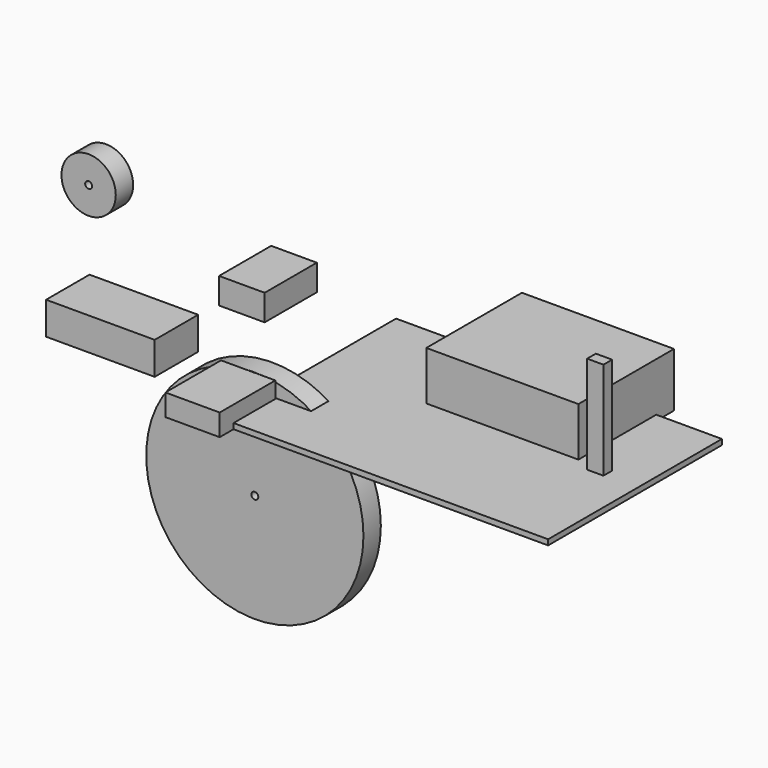
from build123d import *

# Parameters (mm, degrees)
F0_W      = 50
F0_H      = 25
F1_DEPTH  = 15
F2_W      = 70
F2_H      = 55
F3_DEPTH  = 25
F4_W      = 21
F4_H      = 12
F5_DEPTH  = 30
F6_W      = 25
F6_H      = 32
F7_DEPTH  = 10
F8_W      = 150
F8_H      = 100
F9_DEPTH  = 2.5
F10_R     = 50
F10_R_2   = 1.5875
F11_DEPTH = 10
F12_R     = 12.5
F12_R_2   = 1.5875
F13_DEPTH = 10
F14_W     = 7.5
F14_H     = 44.9961
F15_DEPTH = 5


# Not quite as in the source:
# - a feature names something its author has since deleted; it is built from what else it names


with BuildPart() as f1:
    # F0 (on Top) → F1 (new body)
    with BuildSketch(Plane.XY):
        with Locations((-111.7799058557, -7.9904274056)):
            Rectangle(F0_W, F0_H)
    extrude(amount=F1_DEPTH)


with BuildPart() as f3:
    # F2 (on Top) → F3 (new body)
    with BuildSketch(Plane.XY):
        with Locations((40.3834730387, 48.0927660437)):
            Rectangle(F2_W, F2_H)
    extrude(amount=F3_DEPTH)


with BuildPart() as f5:
    # F4 (on Front) → F5 (new body)
    with BuildSketch(Plane.XZ):
        with Locations((-39.0541495681, 50.8754973734)):
            Rectangle(F4_W, F4_H)
    extrude(amount=F5_DEPTH)


with BuildPart() as f7:
    # F6 (on Top) → F7 (new body)
    with BuildSketch(Plane.XY):
        with Locations((-51.6924057156, -26.56879695)):
            Rectangle(F6_W, F6_H)
    extrude(amount=F7_DEPTH)


with BuildPart() as f9:
    # F8 (on Top) → F9 (new body)
    with BuildSketch(Plane.XY):
        with Locations((30.6242685765, 15.3774665831)):
            Rectangle(F8_W, F8_H)
    extrude(amount=F9_DEPTH)


with BuildPart() as f11:
    # F10 (on Front) → F11 (new body)
    with BuildSketch(Plane.XZ):
        with Locations((-49.077399075, -40.1809364557)):
            Circle(F10_R)
        with Locations((-49.077399075, -40.1809364557)):
            Circle(F10_R_2, mode=Mode.SUBTRACT)
    extrude(amount=F11_DEPTH)


with BuildPart() as f13:
    # F12 (on Front) → F13 (new body)
    with BuildSketch(Plane.XZ):
        with Locations((-125.5905777216, 60.8639121056)):
            Circle(F12_R)
        with Locations((-125.5905777216, 60.8639121056)):
            Circle(F12_R_2, mode=Mode.SUBTRACT)
    extrude(amount=F13_DEPTH)


with BuildPart() as f15:
    # F14 (on Front) → F15 (new body)
    with BuildSketch(Plane.XZ):
        with Locations((103.637938503, 39.2873273231)):
            Rectangle(F14_W, F14_H)
    extrude(amount=F15_DEPTH)


solid = Compound([f1.part, f3.part, f5.part, f7.part, f9.part, f11.part, f13.part, f15.part])
